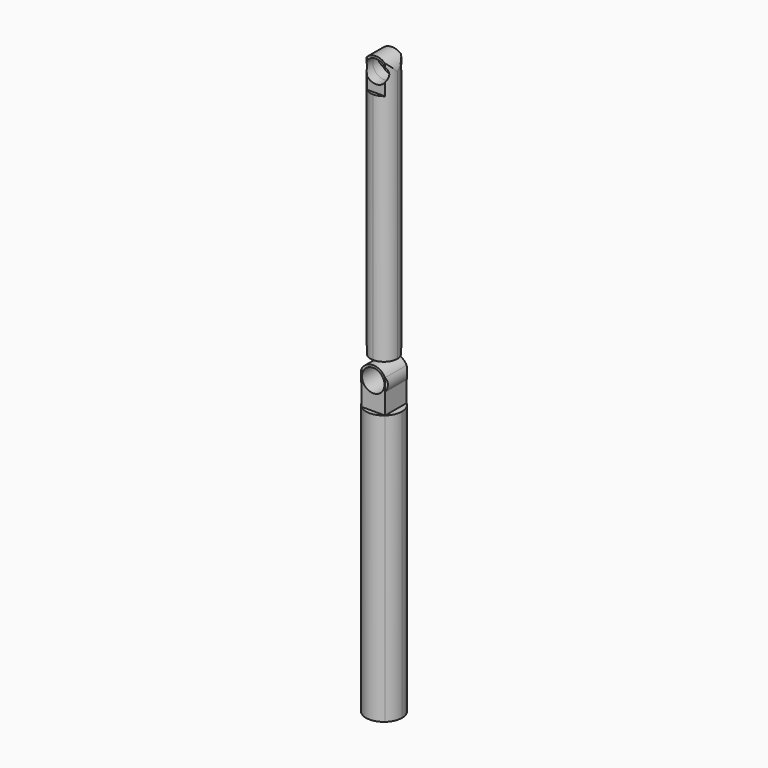
from build123d import *

# Parameters (mm, degrees)
F1_DEPTH  = 70
F2_DEPTH  = 60
F3_DEPTH  = 12
F4_DEPTH  = 10
F5_R      = 2.5
F6_DEPTH  = 25
F8_DEPTH  = 8
F9_R      = 2.5
F10_DEPTH = 12.5


with BuildPart() as f1:
    # F0 (on Top) → F1 (new body)
    with BuildSketch(Plane.XY):
        with BuildLine():
            ThreePointArc((2.6457513111, -3), (3.6457513111, -1.6457513111), (4, 0))
            ThreePointArc((4, 0), (3.6457513111, 1.6457513111), (2.6457513111, 3))
            Line((2.6457513111, 3), (0, 3))
            ThreePointArc((0, 3), (2.1213203436, 2.1213203436), (3, 0))
            ThreePointArc((3, 0), (2.1213203436, -2.1213203436), (0, -3))
            Line((0, -3), (2.6457513111, -3))
        make_face()
        with BuildLine():
            Line((0, 3), (2.6457513111, 3))
            ThreePointArc((2.6457513111, 3), (0, 4), (-2.6457513111, 3))
            Line((-2.6457513111, 3), (0, 3))
        make_face()
        with BuildLine():
            ThreePointArc((-2.6457513111, -3), (0, -4), (2.6457513111, -3))
            Line((2.6457513111, -3), (0, -3))
            Line((0, -3), (-2.6457513111, -3))
        make_face()
        with BuildLine():
            Line((0, 3), (-2.6457513111, 3))
            ThreePointArc((-2.6457513111, 3), (-4, 0), (-2.6457513111, -3))
            Line((-2.6457513111, -3), (0, -3))
            ThreePointArc((0, -3), (-3, 0), (0, 3))
        make_face()
    extrude(amount=-F1_DEPTH)



with BuildPart() as f2:
    # F0 (on Top) → F2 (new body)
    with BuildSketch(Plane.XY):
        with BuildLine():
            ThreePointArc((3, 0), (2.1213203436, 2.1213203436), (0, 3))
            ThreePointArc((0, 3), (-3, 0), (0, -3))
            ThreePointArc((0, -3), (2.1213203436, -2.1213203436), (3, 0))
        make_face()
    extrude(amount=F2_DEPTH)


with BuildPart() as f1_1:
    add(f1.part)

    add(f2.part)  # F3 merges F2
    # F0 (on Top) → F3 (join)
    with BuildSketch(Plane.XY):
        with BuildLine():
            ThreePointArc((3, 0), (2.1213203436, 2.1213203436), (0, 3))
            ThreePointArc((0, 3), (-3, 0), (0, -3))
            ThreePointArc((0, -3), (2.1213203436, -2.1213203436), (3, 0))
        make_face()
    extrude(amount=-F3_DEPTH)

    # F0 (on Top) → F4 (cut)
    with BuildSketch(Plane.XY):
        with BuildLine():
            Line((0, 3), (2.6457513111, 3))
            ThreePointArc((2.6457513111, 3), (0, 4), (-2.6457513111, 3))
            Line((-2.6457513111, 3), (0, 3))
        make_face()
        with BuildLine():
            ThreePointArc((-2.6457513111, -3), (0, -4), (2.6457513111, -3))
            Line((2.6457513111, -3), (0, -3))
            Line((0, -3), (-2.6457513111, -3))
        make_face()
    extrude(amount=-F4_DEPTH, mode=Mode.SUBTRACT)

    # F5 (on face) → F6 (cut)
    with BuildSketch(Plane(origin=(0, 3, 0), x_dir=(-1, 0, 0), z_dir=(0, 1, 0))):
        with Locations((0, -4.0064705536)):
            Circle(F5_R)
        with BuildLine():
            ThreePointArc((-2.6457513111, -5.420684116), (-3, -4.0064705536), (-2.6457513111, -2.5922569912))
            Line((-2.6457513111, -2.5922569912), (-2.6457513111, 0))
            Line((-2.6457513111, 0), (-4, 0))
            Line((-4, 0), (-4, -10))
            Line((-4, -10), (-2.6457513111, -10))
            Line((-2.6457513111, -10), (-2.6457513111, -5.420684116))
        make_face()
        with BuildLine():
            ThreePointArc((2.6457513111, -2.5922569912), (2.9100905427, -3.2775171714), (3, -4.0064705536))
            ThreePointArc((3, -4.0064705536), (2.9100905427, -4.7354239358), (2.6457513111, -5.420684116))
            Line((2.6457513111, -5.420684116), (2.6457513111, -10))
            Line((2.6457513111, -10), (4, -10))
            Line((4, -10), (4, 0))
            Line((4, 0), (2.6457513111, 0))
            Line((2.6457513111, 0), (2.6457513111, -2.5922569912))
        make_face()
        with BuildLine():
            ThreePointArc((-2.6457513111, -2.5922569912), (0, -1.0064705536), (2.6457513111, -2.5922569912))
            Line((2.6457513111, -2.5922569912), (2.6457513111, 0))
            Line((2.6457513111, 0), (1.3542486889, 0))
            Line((1.3542486889, 0), (0, 0))
            Line((0, 0), (-1.3542486889, 0))
            Line((-1.3542486889, 0), (-2.6457513111, 0))
            Line((-2.6457513111, 0), (-2.6457513111, -2.5922569912))
        make_face()
    extrude(amount=-F6_DEPTH, mode=Mode.SUBTRACT)

    # F7 (on face) → F8 (cut)
    with BuildSketch(Plane.XY.offset(60)):
        with BuildLine():
            ThreePointArc((2, 2.2360679775), (0, 3), (-2, 2.2360679775))
            Line((-2, 2.2360679775), (2, 2.2360679775))
        make_face()
        with BuildLine():
            ThreePointArc((-2, -2.2360679775), (0, -3), (2, -2.2360679775))
            Line((2, -2.2360679775), (-2, -2.2360679775))
        make_face()
    extrude(amount=-F8_DEPTH, mode=Mode.SUBTRACT)

    # F9 (on Front) → F10 (cut, symmetric)
    with BuildSketch(Plane.XZ):
        with Locations((0, 56.2073551118)):
            Circle(F9_R)
        with BuildLine():
            Line((-3, 60), (-3, 56.2073551118))
            ThreePointArc((-3, 56.2073551118), (0, 59.2073551118), (3, 56.2073551118))
            Line((3, 56.2073551118), (3, 60))
            Line((3, 60), (-3, 60))
        make_face()
    extrude(amount=F10_DEPTH, both=True, mode=Mode.SUBTRACT)


solid = f1_1.part
